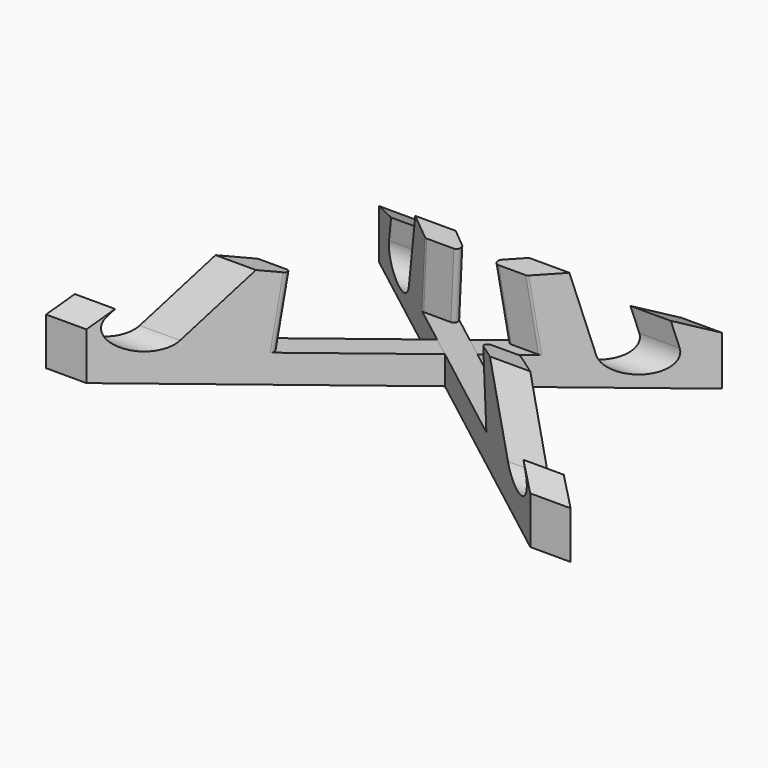
from build123d import *

# Parameters (mm, degrees)
F1_DEPTH      = 25
F2_DEPTH      = 25
F4_DEPTH      = 65.001
F4_DEPTH_BACK = 65.001
F5_DEPTH      = 3.5
F7_R          = 1
F7_2_R        = 1


# Not quite as in the source:
# - a feature of the source that left no trace in its solid (it failed there, or was rolled back) is left out


with BuildPart() as f1:
    # F0 (on Top) → F1 (new body)
    with BuildSketch(Plane.XY):
        Polygon((-65, 0), (-55, 0), (0, 42.3076923077), (-5, 46.1538461538), align=None)
        Polygon((-5, 46.1538461538), (0, 42.3076923077), (5, 46.1538461538), (0, 50), align=None)
        Polygon((0, 50), (5, 46.1538461538), (42.5, 75), (32.5, 75), align=None)
    extrude(amount=F1_DEPTH)


with BuildPart() as f2:
    # F0 (on Top) → F2 (new body)
    with BuildSketch(Plane.XY):
        Polygon((5, 46.1538461538), (0, 42.3076923077), (55, 0), (65, 0), align=None)
        Polygon((-42.5, 75), (-5, 46.1538461538), (0, 50), (-32.5, 75), align=None)
        Polygon((-5, 46.1538461538), (0, 42.3076923077), (5, 46.1538461538), (0, 50), align=None)
    extrude(amount=F2_DEPTH)


with BuildPart() as f4_tool:
    # F3 (on Right) → F4 (new body, two sides)
    with BuildSketch(Plane.YZ) as f4_sk:
        with BuildLine():
            Line((75, 25), (57, 25))
            Line((57, 25), (60.1634270419, 7.0593137296))
            ThreePointArc((60.1634270419, 7.0593137296), (65.9557066953, 3.0035158528), (70.011504572, 8.7957955062))
            Line((70.011504572, 8.7957955062), (68.969615506, 14.7046420243))
            Line((68.969615506, 14.7046420243), (75, 12.2137521295))
            Line((75, 12.2137521295), (75, 25))
        make_face()
        Polygon((57, 25), (20, 25), (25, 24.2972958265), (23.4866827055, 7), (53.5133172945, 7), (52, 24.2972958265), align=None)
        with BuildLine():
            Line((0, 11.7226943725), (3.390477077, 16.2314624079))
            Line((3.390477077, 16.2314624079), (2.390477077, 14.4994116003))
            ThreePointArc((2.390477077, 14.4994116003), (4.2206040959, 7.6692845814), (11.0507311148, 9.4994116003))
            Line((11.0507311148, 9.4994116003), (20, 25))
            Line((20, 25), (0, 25))
            Line((0, 25), (0, 11.7226943725))
        make_face()
    extrude(amount=F4_DEPTH)
    extrude(f4_sk.sketch, amount=-F4_DEPTH_BACK)


with BuildPart() as f1_1:
    add(f1.part)

    # F4: cut by f4_tool
    add(f4_tool.part, mode=Mode.SUBTRACT)


with BuildPart() as f2_1:
    add(f2.part)

    # F4: cut by f4_tool
    add(f4_tool.part, mode=Mode.SUBTRACT)

    # F0 (on Top) → F5 (cut)
    with BuildSketch(Plane.XY):
        Polygon((-5, 46.1538461538), (0, 42.3076923077), (5, 46.1538461538), (0, 50), align=None)
    extrude(amount=F5_DEPTH, mode=Mode.SUBTRACT)


with BuildPart() as f1_2:
    add(f1_1.part)

    # F6: cut F2
    add(f2_1.part, mode=Mode.SUBTRACT)

    # F7
    f7_edges = [f1_2.edges().sort_by_distance(p)[0] for p in [
        (-23.483656, 24.243341, 15.648648),
        (-33.483656, 24.243341, 15.648648),
        (3.583656, 52.756659, 15.648648),
        (13.583656, 52.756659, 15.648648),
    ]]
    fillet(f7_edges, radius=F7_R)


with BuildPart() as f2_2:
    add(f2_1.part)

    # F7#2
    f7_2_edges = [f2_2.edges().sort_by_distance(p)[0] for p in [
        (23.483656, 24.243341, 15.648648),
        (33.483656, 24.243341, 15.648648),
        (-13.583656, 52.756659, 15.648648),
        (-3.583656, 52.756659, 15.648648),
    ]]
    fillet(f7_2_edges, radius=F7_2_R)


solid = Compound([f1_2.part, f2_2.part])
